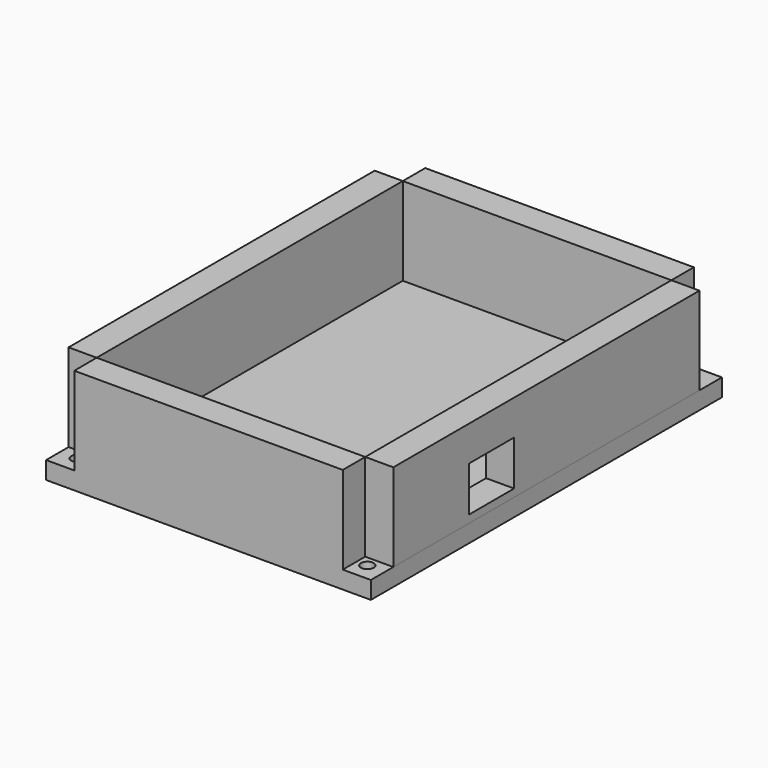
from build123d import *

# Parameters (mm, degrees)
F0_R     = 2.3114
F0_W     = 97.1493866
F0_H     = 10.16
F1_DEPTH = 6.35
F2_DEPTH = 31.75
F3_DEPTH = 31.75
F4_DEPTH = 31.75
F5_DEPTH = 31.75
F7_DEPTH = 10.16


# Not quite as in the source:
# - a feature names something its author has since deleted; it is built from what else it names


with BuildPart() as f1:
    # F0 (on Top) → F1 (new body)
    with BuildSketch(Plane.XY):
        Polygon((12.0852296243, 64.2014063512), (-85.0641569757, 64.2014063512), (-85.0641569757, 61.6614063512), (-85.0641569757, 48.9614063512), (-85.0641569757, -61.5127440488), (-85.0641569757, -74.2127440488), (-72.3641569757, -74.2127440488), (-0.6147703757, -74.2127440488), (12.0852296243, -74.2127440488), (12.0852296243, -61.5127440488), (12.0852296243, 48.9614063512), (12.0852296243, 61.6614063512), align=None)
        Polygon((22.2452296243, -78.0227440488), (22.2452296243, -74.2127440488), (12.0852296243, -74.2127440488), (12.0852296243, -84.3727440488), (15.8952296243, -84.3727440488), (22.2452296243, -84.3727440488), align=None)
        with Locations((15.8952296243, -78.0227440488)):
            Circle(F0_R, mode=Mode.SUBTRACT)
        Polygon((-88.8741569757, 74.3614063512), (-95.2241569757, 74.3614063512), (-95.2241569757, 68.0114063512), (-95.2241569757, 64.2014063512), (-85.0641569757, 64.2014063512), (-85.0641569757, 74.3614063512), align=None)
        with Locations((-88.8741569757, 68.0114063512)):
            Circle(F0_R, mode=Mode.SUBTRACT)
        Polygon((-85.0641569757, -74.2127440488), (-95.2241569757, -74.2127440488), (-95.2241569757, -78.0227440488), (-95.2241569757, -84.3727440488), (-88.8741569757, -84.3727440488), (-85.0641569757, -84.3727440488), (-85.026336457, -84.3727440488), align=None)
        with Locations((-88.8741569757, -78.0227440488)):
            Circle(F0_R, mode=Mode.SUBTRACT)
        Polygon((22.2452296243, 64.2014063512), (12.0852296243, 64.2014063512), (12.0852296243, 61.6614063512), (12.0852296243, 48.9614063512), (12.0852296243, -61.5127440488), (12.0852296243, -74.2127440488), (22.2452296243, -74.2127440488), align=None)
        Polygon((-72.3641569757, -74.2127440488), (-85.0641569757, -74.2127440488), (-85.026336457, -84.3727440488), (12.0852296243, -84.3727440488), (12.0852296243, -74.2127440488), (-0.6147703757, -74.2127440488), align=None)
        with Locations((-36.4894636757, 69.2814063512)):
            Rectangle(F0_W, F0_H)
        Polygon((-85.0641569757, 64.2014063512), (-95.2241569757, 64.2014063512), (-95.2241569757, 61.6614063512), (-95.2241569757, -74.2127440488), (-85.0641569757, -74.2127440488), (-85.0641569757, -61.5127440488), (-85.0641569757, 48.9614063512), (-85.0641569757, 61.6614063512), align=None)
        Polygon((15.8952296243, 74.3614063512), (12.0852296243, 74.3614063512), (12.0852296243, 64.2014063512), (22.2452296243, 64.2014063512), (22.2452296243, 68.0114063512), (22.2452296243, 74.3614063512), align=None)
        with Locations((15.8952296243, 68.0114063512)):
            Circle(F0_R, mode=Mode.SUBTRACT)
    extrude(amount=-F1_DEPTH)

    # F0 (on Top) → F2 (join)
    with BuildSketch(Plane.XY):
        with Locations((-36.4894636757, 69.2814063512)):
            Rectangle(F0_W, F0_H)
    extrude(amount=F2_DEPTH)

    # F0 (on Top) → F3 (join)
    with BuildSketch(Plane.XY):
        Polygon((-72.3641569757, -74.2127440488), (-85.0641569757, -74.2127440488), (-85.026336457, -84.3727440488), (12.0852296243, -84.3727440488), (12.0852296243, -74.2127440488), (-0.6147703757, -74.2127440488), align=None)
    extrude(amount=F3_DEPTH)


with BuildPart() as f4:
    # F0 (on Top) → F4 (new body)
    with BuildSketch(Plane.XY):
        Polygon((22.2452296243, 64.2014063512), (12.0852296243, 64.2014063512), (12.0852296243, 61.6614063512), (12.0852296243, 48.9614063512), (12.0852296243, -61.5127440488), (12.0852296243, -74.2127440488), (22.2452296243, -74.2127440488), align=None)
    extrude(amount=F4_DEPTH)

    # F6 (on face) → F7 (cut)
    with BuildSketch(Plane.YZ.offset(22.2452296243)):
        Polygon((-39.9227440488, 19.05), (-39.9227440488, 17.3254348338), (-39.9227440488, 2.794), (-19.6027440488, 2.794), (-19.6027440488, 19.05), (-31.9871492684, 19.05), align=None)
    extrude(amount=-F7_DEPTH, mode=Mode.SUBTRACT)


with BuildPart() as f5:
    # F0 (on Top) → F5 (new body)
    with BuildSketch(Plane.XY):
        Polygon((-85.0641569757, 64.2014063512), (-95.2241569757, 64.2014063512), (-95.2241569757, 61.6614063512), (-95.2241569757, -74.2127440488), (-85.0641569757, -74.2127440488), (-85.0641569757, -61.5127440488), (-85.0641569757, 48.9614063512), (-85.0641569757, 61.6614063512), align=None)
    extrude(amount=F5_DEPTH)


solid = Compound([f1.part, f4.part, f5.part])
